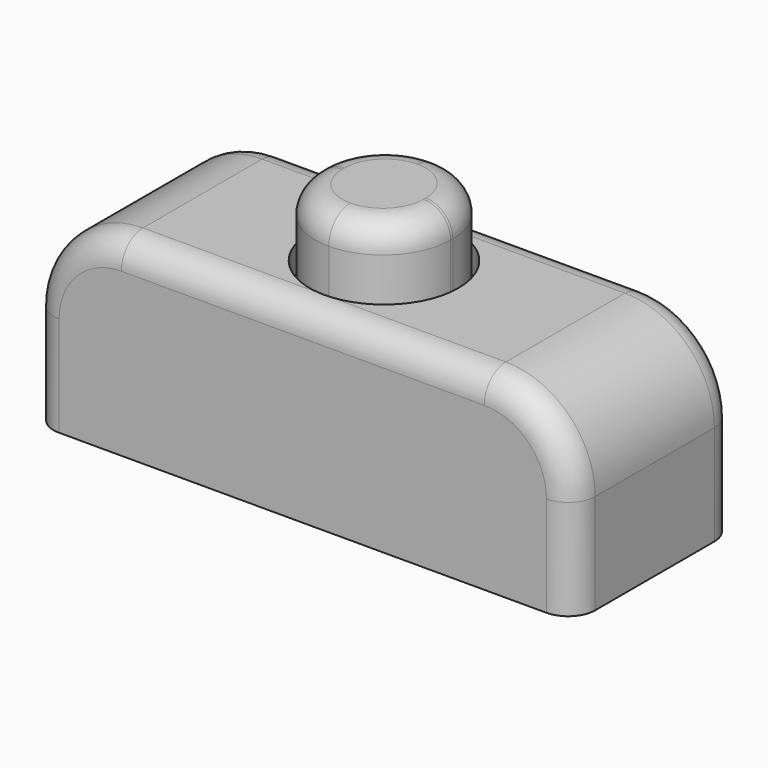
from build123d import *

# Parameters (mm, degrees)
F0_W     = 50.8
F0_H     = 19.05
F0_W_2   = 45.72
F0_H_2   = 13.97
F1_DEPTH = 12.7
F2_W     = 50.8
F2_H     = 19.05
F3_DEPTH = 2.54
F5_START = 0.508
F4_W     = 4.572
F4_H     = 2.794
F4_W_2   = 12.7
F4_H_2   = 5.08
F4_H_3   = 3.81
F5_DEPTH = 12.954
F6_R     = 6.34999
F7_W     = 50.8
F7_H     = 19.05
F7_R     = 6.985
F8_DEPTH = 2.54
F9_R     = 2.54
F10_R    = 8.382
F11_R    = 2.54


# Not quite as in the source:
# - a fillet or chamfer is up to 0.001 mm smaller than in the source, because OpenCascade refuses the exact size


with BuildPart() as f1:
    # F0 (on Top) → F1 (new body)
    with BuildSketch(Plane.XY):
        Rectangle(F0_W, F0_H)
        Rectangle(F0_W_2, F0_H_2, mode=Mode.SUBTRACT)
    extrude(amount=F1_DEPTH)

    # F2 (on face) → F3 (join)
    with BuildSketch(Plane(origin=(0, 0, 0), x_dir=(1, 0, 0), z_dir=(0, 0, -1))):
        Rectangle(F2_W, F2_H)
    extrude(amount=F3_DEPTH)

    # F4 (on face) → F5 (join)
    with BuildSketch(Plane.XZ.offset(-6.985).offset(F5_START)):
        Polygon((-25.4, 0.254), (-25.4, -2.54), (20.828, -2.54), (20.828, 0.254), (-20.828, 0.254), align=None)
        with Locations((23.114, -1.143)):
            Rectangle(F4_W, F4_H)
        with BuildLine():
            Line((-20.828, 0.254), (20.828, 0.254))
            Line((20.828, 0.254), (20.828, 0.508))
            ThreePointArc((20.828, 0.508), (19.7166563034, 0.9891715443), (19.3070802744, 2.1288462099))
            Line((19.3070802744, 2.1288462099), (5.08, 7.62))
            Line((5.08, 7.62), (-5.08, 7.62))
            Line((-5.08, 7.62), (-19.3070802744, 2.1288462099))
            ThreePointArc((-19.3070802744, 2.1288462099), (-19.3047702633, 2.0804475914), (-19.304, 2.032))
            ThreePointArc((-19.304, 2.032), (-19.7503692655, 0.9543692655), (-20.828, 0.508))
            Line((-20.828, 0.508), (-20.828, 0.254))
        make_face()
        with BuildLine():
            ThreePointArc((19.3070802744, 2.1288462099), (19.7166563034, 0.9891715443), (20.828, 0.508))
            Line((20.828, 0.508), (20.828, 2.032))
            Line((20.828, 2.032), (19.558, 2.032))
            Line((19.558, 2.032), (19.3070802744, 2.1288462099))
        make_face()
        with BuildLine():
            Line((20.828, 2.032), (20.828, 0.508))
            ThreePointArc((20.828, 0.508), (21.9056307345, 0.9543692655), (22.352, 2.032))
            ThreePointArc((22.352, 2.032), (21.7251962822, 3.2639151071), (20.3603794867, 3.4824851104))
            Line((20.3603794867, 3.4824851104), (20.828, 3.302))
            Line((20.828, 3.302), (20.828, 2.032))
        make_face()
        with BuildLine():
            ThreePointArc((-20.3603794867, 3.4824851104), (-22.3335091013, 2.2686819509), (-20.828, 0.508))
            Line((-20.828, 0.508), (-20.828, 2.032))
            Line((-20.828, 2.032), (-20.828, 3.302))
            Line((-20.828, 3.302), (-20.3603794867, 3.4824851104))
        make_face()
        with BuildLine():
            Line((-20.828, 2.032), (-20.828, 0.508))
            ThreePointArc((-20.828, 0.508), (-19.7503692655, 0.9543692655), (-19.304, 2.032))
            ThreePointArc((-19.304, 2.032), (-19.3047702633, 2.0804475914), (-19.3070802744, 2.1288462099))
            Line((-19.3070802744, 2.1288462099), (-19.558, 2.032))
            Line((-19.558, 2.032), (-20.828, 2.032))
        make_face()
        with BuildLine():
            Line((19.558, 2.032), (20.828, 2.032))
            Line((20.828, 2.032), (20.828, 3.302))
            Line((20.828, 3.302), (20.3603794867, 3.4824851104))
            ThreePointArc((20.3603794867, 3.4824851104), (19.6252291828, 2.9679051027), (19.3070802744, 2.1288462099))
            Line((19.3070802744, 2.1288462099), (19.558, 2.032))
        make_face()
        with BuildLine():
            Line((5.08, 7.62), (19.3070802744, 2.1288462099))
            ThreePointArc((19.3070802744, 2.1288462099), (19.6252291828, 2.9679051027), (20.3603794867, 3.4824851104))
            Line((20.3603794867, 3.4824851104), (6.35, 8.89))
            Line((6.35, 8.89), (6.35, 7.62))
            Line((6.35, 7.62), (5.08, 7.62))
        make_face()
        with BuildLine():
            Line((-20.828, 3.302), (-20.828, 2.032))
            Line((-20.828, 2.032), (-19.558, 2.032))
            Line((-19.558, 2.032), (-19.3070802744, 2.1288462099))
            ThreePointArc((-19.3070802744, 2.1288462099), (-19.6252291828, 2.9679051027), (-20.3603794867, 3.4824851104))
            Line((-20.3603794867, 3.4824851104), (-20.828, 3.302))
        make_face()
        with BuildLine():
            Line((-6.35, 8.89), (-20.3603794867, 3.4824851104))
            ThreePointArc((-20.3603794867, 3.4824851104), (-19.6252291828, 2.9679051027), (-19.3070802744, 2.1288462099))
            Line((-19.3070802744, 2.1288462099), (-5.08, 7.62))
            Line((-5.08, 7.62), (-6.35, 7.62))
            Line((-6.35, 7.62), (-6.35, 8.89))
        make_face()
        Polygon((-5.08, 7.62), (5.08, 7.62), (6.35, 7.62), (6.35, 8.89), (6.35, 12.7), (-6.35, 12.7), (-6.35, 8.89), (-6.35, 7.62), align=None)
        with Locations((0, 15.24)):
            Rectangle(F4_W_2, F4_H_2)
        with Locations((0, 19.685)):
            Rectangle(F4_W_2, F4_H_3)
    extrude(amount=F5_DEPTH)

    # F6 (radius 6.35 in the source; OpenCascade refuses exactly that, so slightly less here)
    f6_edges = [f1.edges().sort_by_distance(p)[0] for p in [
        (-6.35, -6.477, 15.24),
        (6.35, -6.477, 15.24),
        (6.35, 6.477, 15.24),
        (-6.35, 6.477, 15.24),
    ]]
    fillet(f6_edges, radius=F6_R)

    # F7 (on face) → F8 (join)
    with BuildSketch(Plane.XY.offset(12.7)):
        Rectangle(F7_W, F7_H)
        Circle(F7_R, mode=Mode.SUBTRACT)
    extrude(amount=F8_DEPTH)

    # F9
    f9_edges = [f1.edges().sort_by_distance(p)[0] for p in [
        (4.490131, -4.617131, 21.59),
    ]]
    fillet(f9_edges, radius=F9_R)

    # F10
    f10_edges = [f1.edges().sort_by_distance(p)[0] for p in [
        (25.4, 0, 15.24),
        (-25.4, 0, 15.24),
    ]]
    fillet(f10_edges, radius=F10_R)

    # F11
    f11_edges = [f1.edges().sort_by_distance(p)[0] for p in [
        (0, 9.525, 15.24),
        (0, -9.525, 15.24),
        (-22.944969, -9.525, 12.784969),
        (-22.944969, 9.525, 12.784969),
        (-25.4, 9.525, 2.159),
        (-25.4, -9.525, 2.159),
        (25.4, 9.525, 2.159),
        (22.944969, 9.525, 12.784969),
        (22.944969, -9.525, 12.784969),
        (25.4, -9.525, 2.159),
    ]]
    fillet(f11_edges, radius=F11_R)


solid = f1.part
